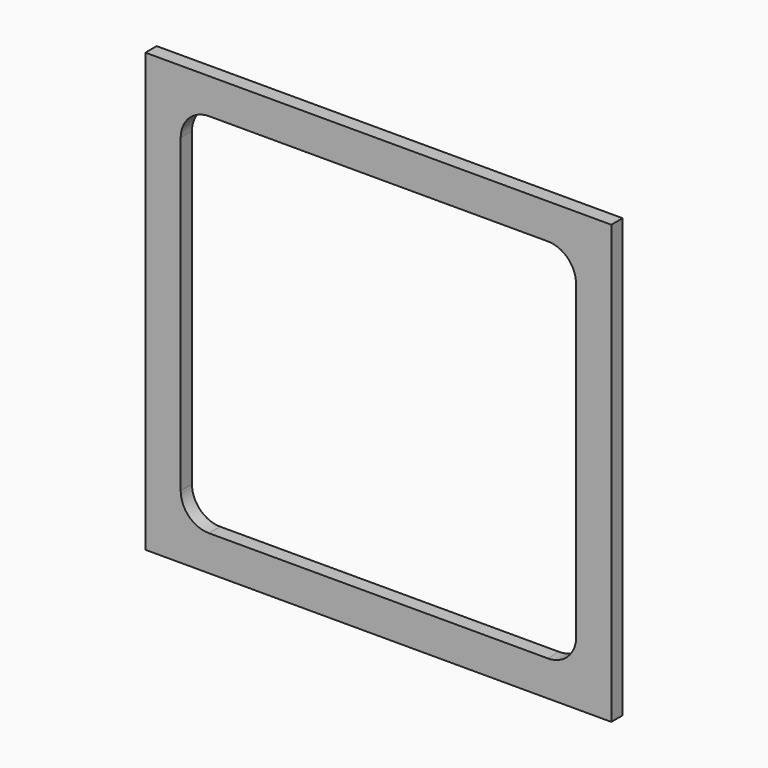
from build123d import *

# Parameters (mm, degrees)
F0_W     = 660
F0_H     = 620
F1_DEPTH = 20


# Not quite as in the source:
# - a feature names something its author has since deleted; it is built from what else it names


with BuildPart() as f1:
    # F0 (on Front) → F1 (new body)
    with BuildSketch(Plane.XZ):
        with Locations((50.7417723536, 80.0849853243)):
            Rectangle(F0_W, F0_H)
        with BuildLine():
            ThreePointArc((-229.2582276464, 300.0849257198), (-217.5423250388, 328.3694304295), (-189.2576763034, 340.0849853243))
            Line((-189.2576763034, 340.0849853243), (290.7423236966, 340.0849853243))
            ThreePointArc((290.7423236966, 340.0849853243), (319.026238531, 328.3690616443), (330.7417723536, 300.0849853241))
            Line((330.7417723536, 300.0849853241), (330.7417723536, -134.9150146759))
            ThreePointArc((330.7417723536, -134.9150146759), (320.9520306177, -166.4907997995), (290.7417723536, -179.9150146759))
            Line((290.7417723536, -179.9150146759), (-189.2582276464, -179.9150146759))
            ThreePointArc((-189.2582276464, -179.9150146759), (-217.5424988938, -168.1992859234), (-229.2582276464, -139.9150146759))
            Line((-229.2582276464, -139.9150146759), (-229.2582276464, 300.0849257198))
        make_face(mode=Mode.SUBTRACT)
    extrude(amount=F1_DEPTH)


solid = f1.part
